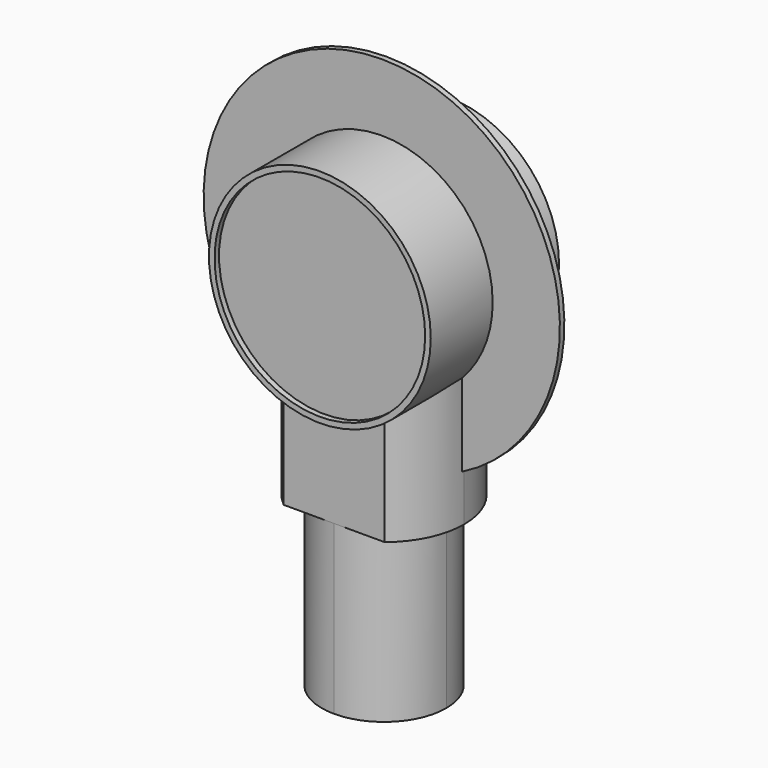
from build123d import *

# Parameters (mm, degrees)
F1_R     = 18.85
F2_DEPTH = 13.35
F1_R_2   = 19.85
F3_DEPTH = 14.35
F4_DEPTH = 34.2
F5_DEPTH = 30
F6_DEPTH = 20.9
F1_R_3   = 31.8850678314
F8_DEPTH = 0.5


with BuildPart() as f2:
    # F1 (on Front) → F2 (new body, symmetric)
    with BuildSketch(Plane.XZ):
        with Locations((0, 36.9661189616)):
            Circle(F1_R)
    extrude(amount=F2_DEPTH, both=True)

    # F1 (on Front) → F3 (join, symmetric)
    with BuildSketch(Plane.XZ):
        with Locations((0, 36.9661189616)):
            Circle(F1_R_2)
        with Locations((0, 36.9661189616)):
            Circle(F1_R, mode=Mode.SUBTRACT)
    extrude(amount=F3_DEPTH, both=True)



with BuildPart() as f4:
    # F0 (on Top) → F4 (new body)
    with BuildSketch(Plane.XY):
        with BuildLine():
            ThreePointArc((5.4e-09, -11.15), (7.8842406121, -7.8842406083), (11.15, 0))
            ThreePointArc((11.15, 0), (7.8842406263, 7.8842405941), (4.56e-08, 11.15))
            ThreePointArc((4.56e-08, 11.15), (-11.15, 2.01e-08), (5.4e-09, -11.15))
        make_face()
        with BuildLine():
            ThreePointArc((4.56e-08, 11.15), (7.8842406263, 7.8842405941), (11.15, 0))
            ThreePointArc((11.15, 0), (7.8842406121, -7.8842406083), (5.4e-09, -11.15))
            Line((5.4e-09, -11.15), (9.0332718325, -11.15))
            ThreePointArc((9.0332718325, -11.15), (12.9527979757, -6.1763682372), (14.35, 0))
            ThreePointArc((14.35, 0), (12.9527979757, 6.1763682372), (9.0332718325, 11.15))
            Line((9.0332718325, 11.15), (4.56e-08, 11.15))
        make_face()
        with BuildLine():
            ThreePointArc((5.4e-09, -11.15), (-11.15, 2.01e-08), (4.56e-08, 11.15))
            Line((4.56e-08, 11.15), (-9.0332718325, 11.15))
            ThreePointArc((-9.0332718325, 11.15), (-12.9527979757, 6.1763682372), (-14.35, 0))
            ThreePointArc((-14.35, 0), (-12.9527979757, -6.1763682372), (-9.0332718325, -11.15))
            Line((-9.0332718325, -11.15), (5.4e-09, -11.15))
        make_face()
    extrude(amount=F4_DEPTH)

    # F0 (on Top) → F5 (join)
    with BuildSketch(Plane.XY):
        with BuildLine():
            ThreePointArc((5.4e-09, -11.15), (7.8842406121, -7.8842406083), (11.15, 0))
            ThreePointArc((11.15, 0), (7.8842406263, 7.8842405941), (4.56e-08, 11.15))
            ThreePointArc((4.56e-08, 11.15), (-11.15, 2.01e-08), (5.4e-09, -11.15))
        make_face()
    extrude(amount=-F5_DEPTH)


with BuildPart() as f6:
    # F1 (on Front) → F6 (new body, symmetric)
    with BuildSketch(Plane.XZ):
        with Locations((0, 36.9661189616)):
            Circle(F1_R_2)
        with Locations((0, 36.9661189616)):
            Circle(F1_R, mode=Mode.SUBTRACT)
        with Locations((0, 36.9661189616)):
            Circle(F1_R)
    extrude(amount=F6_DEPTH, both=True)


with BuildPart() as f4_1:
    add(f4.part)

    # F7: cut F6
    add(f6.part, mode=Mode.SUBTRACT)


with BuildPart() as f2_1:
    add(f2.part)

    add(f4_1.part)  # F8 merges F4
    # F1 (on Front) → F8 (join, symmetric)
    with BuildSketch(Plane.XZ):
        with Locations((0, 36.9661189616)):
            Circle(F1_R_3)
        with Locations((0, 36.9661189616)):
            Circle(F1_R_2, mode=Mode.SUBTRACT)
    extrude(amount=F8_DEPTH, both=True)


solid = f2_1.part
